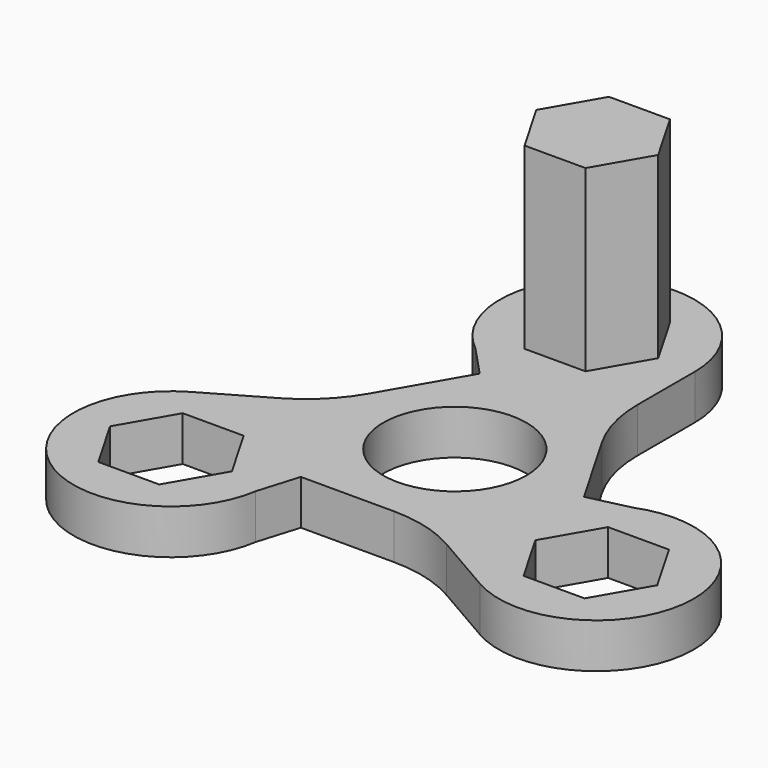
from build123d import *

# Parameters (mm, degrees)
F0_R     = 8
F1_DEPTH = 5
F2_DEPTH = 5
F3_COUNT = 3
F4_DEPTH = 25
F5_R     = 15


# Not quite as in the source:
# - a feature names something its author has since deleted; it is built from what else it names


with BuildPart() as f1:
    # F0 (on Top) → F1 (new body)
    with BuildSketch(Plane.XY):
        Polygon((7.2168783649, 12.5), (-7.2168783649, 12.5), (-14.4337567297, 0), (-7.2168783649, -12.5), (7.2168783649, -12.5), (14.4337567297, 0), align=None)
        Circle(F0_R, mode=Mode.SUBTRACT)
    extrude(amount=F1_DEPTH)

    # F0 (on Top) → F2 (join)
    with BuildSketch(Plane.XY):
        with BuildLine():
            Line((-10.4958548116, 15.991376923), (-7.2168783649, 12.5))
            Line((-7.2168783649, 12.5), (7.2168783649, 12.5))
            Line((7.2168783649, 12.5), (7.2168783649, 24.5))
            ThreePointArc((7.2168783649, 24.5), (-8.4028254594, 34.3251918969), (-10.4958548116, 15.991376923))
        make_face()
        Polygon((-10.4958548116, 24.5), (-7.0894882233, 30.4), (-0.2767550469, 30.4), (3.1296115413, 24.5), (-0.2767550469, 18.6), (-7.0894882233, 18.6), align=None, mode=Mode.SUBTRACT)
    extrude(amount=F2_DEPTH)

    # F3: F1 ×3 about axis
    f3_axis = Axis((0, 0, 0), (0, 0, 1))


with BuildPart() as f1_1:
    add(f1.part)
    for i in range(1, F3_COUNT):
        add(f1.part.rotate(f3_axis, i * 360 / F3_COUNT))

    # F5
    f5_edges = [f1_1.edges().sort_by_distance(p)[0] for p in [
        (7.216878, 12.5, 2.5),
        (7.216878, -12.5, 2.5),
        (-14.433757, 0, 2.5),
    ]]
    fillet(f5_edges, radius=F5_R)


with BuildPart() as f4:
    # F0 (on Top) → F4 (new body)
    with BuildSketch(Plane.XY):
        Polygon((-0.2767550469, 30.4), (-7.0894882233, 30.4), (-10.4958548116, 24.5), (-7.0894882233, 18.6), (-0.2767550469, 18.6), (3.1296115413, 24.5), align=None)
    extrude(amount=F4_DEPTH)


solid = Compound([f1_1.part, f4.part])
